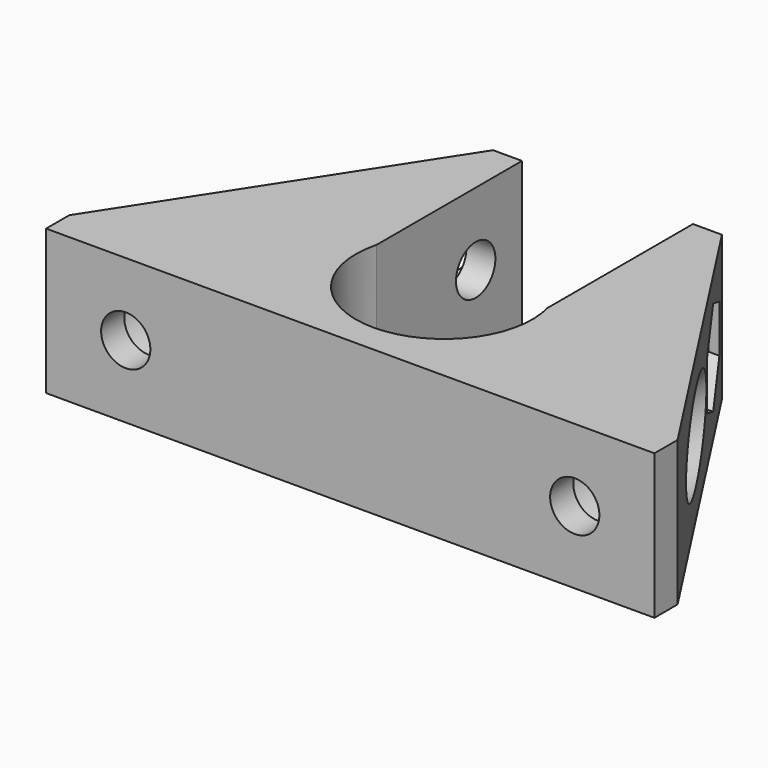
from build123d import *

# Parameters (mm, degrees)
F1_DEPTH      = 5
F2_R          = 1.7
F3_DEPTH      = 22.201
F5_R          = 3
F6_DEPTH      = 20.201
F7_R          = 1.7
F8_DEPTH      = 21.001
F8_DEPTH_BACK = 21.001
F11_DEPTH     = 13.101


# Not quite as in the source:
# - a pattern or mirror of a feature is missing from the dataset's text; its kind, count and spacing are read off the source's solid


with BuildPart() as f1:
    # F0 (on Top) → F1 (new body, symmetric)
    with BuildSketch(Plane.XY):
        with BuildLine():
            Line((-21, 2), (-21, 0))
            Line((-21, 0), (21, 0))
            Line((21, 0), (21, 2))
            Line((21, 2), (7.9, 22.2))
            Line((7.9, 22.2), (5.9, 22.2))
            Line((5.9, 22.2), (5.9, 9.6491933385))
            ThreePointArc((5.9, 9.6491933385), (0, 2), (-5.9, 9.6491933385))
            Line((-5.9, 9.6491933385), (-5.9, 22.2))
            Line((-5.9, 22.2), (-7.9, 22.2))
            Line((-7.9, 22.2), (-21, 2))
        make_face()
    extrude(amount=F1_DEPTH, both=True)

    # F2 (on Front) → F3 (cut, through all)
    with BuildSketch(Plane.XZ):
        with Locations((-15.5, 0)):
            Circle(F2_R)
        with Locations((15.5, 0)):
            Circle(F2_R)
    extrude(amount=-F3_DEPTH, mode=Mode.SUBTRACT)

    # F5 (on plane+point) → F6 (cut, through all)
    with BuildSketch(Plane.XZ.offset(-2)):
        with Locations((-15.5, 0)):
            Circle(F5_R)
        with Locations((15.5, 0)):
            Circle(F5_R)
    extrude(amount=-F6_DEPTH, mode=Mode.SUBTRACT)

    # F7 (on Right) → F8 (cut, two sides)
    with BuildSketch(Plane.YZ) as f8_sk:
        with Locations((18.2, 0)):
            Circle(F7_R)
    extrude(amount=-F8_DEPTH, mode=Mode.SUBTRACT)
    extrude(f8_sk.sketch, amount=F8_DEPTH_BACK, mode=Mode.SUBTRACT)

    # F10 (on plane+point) → F11 (cut, through all)
    with BuildSketch(Plane.YZ.offset(7.9)):
        Polygon((18.2, -3.2908965344), (21.05, -1.6454482672), (21.05, 1.6454482672), (18.2, 3.2908965344), (15.35, 1.6454482672), (15.35, -1.6454482672), align=None)
    f11 = extrude(amount=F11_DEPTH, mode=Mode.SUBTRACT)

    # F11_copies: F11 across plane
    add(f11.mirror(Plane(origin=(0, 0, 0), x_dir=(0, 0, -1), z_dir=(-1, 0, 0))), mode=Mode.SUBTRACT)


solid = f1.part
